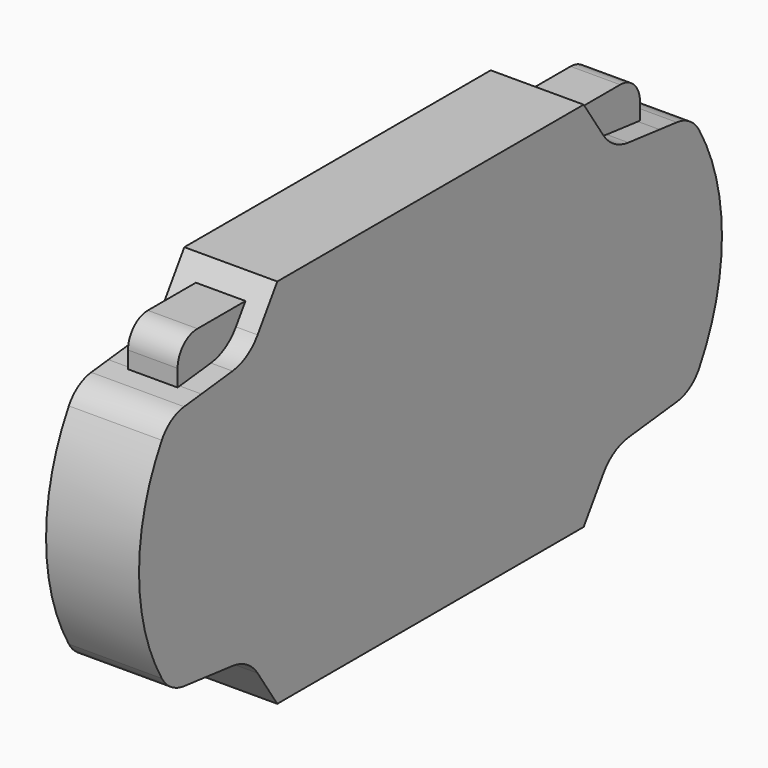
from build123d import *

# Parameters (mm, degrees)
F1_DEPTH  = 7.5
F3_DEPTH  = 4
F5_R      = 3.5
F6_DEPTH  = 3
F7_R      = 5
F8_DEPTH  = 2
F4_W      = 60
F4_H      = 35
F10_DEPTH = 2


# Not quite as in the source:
# - a fillet or chamfer that OpenCascade refuses, or shapes differently, is made with other operations: its cross-section is extruded or revolved along the edge and cut away or added


with BuildPart() as f1:
    # F0 (on Right) → F1 (new body, symmetric)
    with BuildSketch(Plane.YZ):
        with BuildLine():
            Line((-34.8711436077, -24.0259013658), (-30.9017617255, -30))
            Line((-30.9017617255, -30), (0, -30))
            Line((0, -30), (0, 0))
            Line((0, 0), (-52.5, 0))
            Line((-52.5, 0), (-52.5, -18.7762488504))
            ThreePointArc((-52.5, -18.7762488504), (-51.1634624835, -19.4917800985), (-49.6902439515, -19.8494736223))
            Line((-49.6902439515, -19.8494736223), (-46.2112579103, -20.2390480822))
            Line((-46.2112579103, -20.2390480822), (-39.9225158206, -20.9432570884))
            ThreePointArc((-39.9225158206, -20.9432570884), (-37.0550608987, -21.9245400717), (-34.8711436077, -24.0259013658))
        make_face()
        with BuildLine():
            Line((0, 0), (0, -30))
            Line((0, -30), (30.9017617255, -30))
            Line((30.9017617255, -30), (34.8711436077, -24.0259013658))
            ThreePointArc((34.8711436077, -24.0259013658), (37.0550608987, -21.9245400717), (39.9225158206, -20.9432570884))
            Line((39.9225158206, -20.9432570884), (46.2112579103, -20.2390480822))
            Line((46.2112579103, -20.2390480822), (49.6902439515, -19.8494736223))
            ThreePointArc((49.6902439515, -19.8494736223), (51.1634624835, -19.4917800985), (52.5, -18.7762488504))
            Line((52.5, -18.7762488504), (52.5, 0))
            Line((52.5, 0), (0, 0))
        make_face()
        with BuildLine():
            Line((-52.5, 0), (0, 0))
            Line((0, 0), (0, 30))
            Line((0, 30), (-30.9017617255, 30))
            Line((-30.9017617255, 30), (-34.8711436077, 24.0259013658))
            ThreePointArc((-34.8711436077, 24.0259013658), (-37.0550608987, 21.9245400717), (-39.9225158206, 20.9432570884))
            Line((-39.9225158206, 20.9432570884), (-46.2112579103, 20.2390480822))
            Line((-46.2112579103, 20.2390480822), (-49.6902439515, 19.8494736223))
            ThreePointArc((-49.6902439515, 19.8494736223), (-51.1634624835, 19.4917800985), (-52.5, 18.7762488504))
            Line((-52.5, 18.7762488504), (-52.5, 0))
        make_face()
        with BuildLine():
            Line((0, 30), (0, 0))
            Line((0, 0), (52.5, 0))
            Line((52.5, 0), (52.5, 18.7762488504))
            ThreePointArc((52.5, 18.7762488504), (51.1634624835, 19.4917800985), (49.6902439515, 19.8494736223))
            Line((49.6902439515, 19.8494736223), (46.2112579103, 20.2390480822))
            Line((46.2112579103, 20.2390480822), (39.9225158206, 20.9432570884))
            ThreePointArc((39.9225158206, 20.9432570884), (37.0550608987, 21.9245400717), (34.8711436077, 24.0259013658))
            Line((34.8711436077, 24.0259013658), (30.9017617255, 30))
            Line((30.9017617255, 30), (0, 30))
        make_face()
        with BuildLine():
            Line((58.7885477615, 0), (52.5, 0))
            Line((52.5, 0), (52.5, -18.7762488504))
            ThreePointArc((52.5, -18.7762488504), (53.448824854, -17.9374222983), (54.2004466552, -16.9181268278))
            ThreePointArc((54.2004466552, -16.9181268278), (57.6211742241, -8.7646119013), (58.7885477615, 0))
        make_face()
        with BuildLine():
            Line((52.5, 18.7762488504), (52.5, 0))
            Line((52.5, 0), (58.7885477615, 0))
            ThreePointArc((58.7885477615, 0), (57.6211742241, 8.7646119013), (54.2004466552, 16.9181268278))
            ThreePointArc((54.2004466552, 16.9181268278), (53.448824854, 17.9374222983), (52.5, 18.7762488504))
        make_face()
        with BuildLine():
            Line((-58.7885477615, 0), (-52.5, 0))
            Line((-52.5, 0), (-52.5, 18.7762488504))
            ThreePointArc((-52.5, 18.7762488504), (-53.448824854, 17.9374222983), (-54.2004466552, 16.9181268278))
            ThreePointArc((-54.2004466552, 16.9181268278), (-57.6211742241, 8.7646119013), (-58.7885477615, 0))
        make_face()
        with BuildLine():
            Line((-52.5, -18.7762488504), (-52.5, 0))
            Line((-52.5, 0), (-58.7885477615, 0))
            ThreePointArc((-58.7885477615, 0), (-57.6211742241, -8.7646119013), (-54.2004466552, -16.9181268278))
            ThreePointArc((-54.2004466552, -16.9181268278), (-53.448824854, -17.9374222983), (-52.5, -18.7762488504))
        make_face()
    extrude(amount=F1_DEPTH, both=True)

    # F2 (on Right) → F3 (join, symmetric)
    with BuildSketch(Plane.YZ):
        with BuildLine():
            Line((29.7115407884, 26.9230790436), (29.7115407884, 18.846154213))
            Line((29.7115407884, 18.846154213), (46.6346181929, 18.846154213))
            Line((46.6346181929, 18.846154213), (46.6346181929, 22.9230790436))
            ThreePointArc((46.6346181929, 22.9230790436), (45.4630453177, 25.7515061684), (42.6346181929, 26.9230790436))
            Line((42.6346181929, 26.9230790436), (29.7115407884, 26.9230790436))
        make_face()
        with BuildLine():
            Line((-29.7115407884, 18.846154213), (-29.7115407884, 26.9230790436))
            Line((-29.7115407884, 26.9230790436), (-42.6346181929, 26.9230790436))
            ThreePointArc((-42.6346181929, 26.9230790436), (-45.4630453177, 25.7515061684), (-46.6346181929, 22.9230790436))
            Line((-46.6346181929, 22.9230790436), (-46.6346181929, 18.846154213))
            Line((-46.6346181929, 18.846154213), (-29.7115407884, 18.846154213))
        make_face()
    extrude(amount=F3_DEPTH, both=True)

    # F5 (on face) → F6 (join)
    with BuildSketch(Plane(origin=(-7.5, 0, 0), x_dir=(0, -1, 0), z_dir=(-1, 0, 0))):
        with Locations((-43.3653853834, -9.6153849736)):
            Circle(F5_R)
    extrude(amount=F6_DEPTH)

    # F7 (on face) → F8 (join)
    with BuildSketch(Plane(origin=(-10.5, 0, 0), x_dir=(0, -1, 0), z_dir=(-1, 0, 0))):
        with Locations((-43.3653853834, -9.6153849736)):
            Circle(F7_R)
    extrude(amount=F8_DEPTH)

    # F9: fillet of radius 5 on 1 edges, made by hand

    # F9_s1 → F9_t2 (revolve, cut)
    with BuildSketch(Plane.XY.offset(-9.6153849736)):
        with BuildLine():
            ThreePointArc((-10.5, 38.3653853834), (-11.972135955, 40.1293174059), (-12.5, 42.3653853834))
            Line((-12.5, 42.3653853834), (-12.5, 38.3653853834))
            Line((-12.5, 38.3653853834), (-10.5, 38.3653853834))
        make_face()
    revolve(axis=Axis((-12.5, 43.3653853834, -9.6153849736), (-1, 0, 0)), mode=Mode.SUBTRACT)

    # F4 (on face) → F10 (cut)
    with BuildSketch(Plane(origin=(-7.5, 0, 0), x_dir=(0, -1, 0), z_dir=(-1, 0, 0))):
        Rectangle(F4_W, F4_H)
    extrude(amount=-F10_DEPTH, mode=Mode.SUBTRACT)


solid = f1.part
